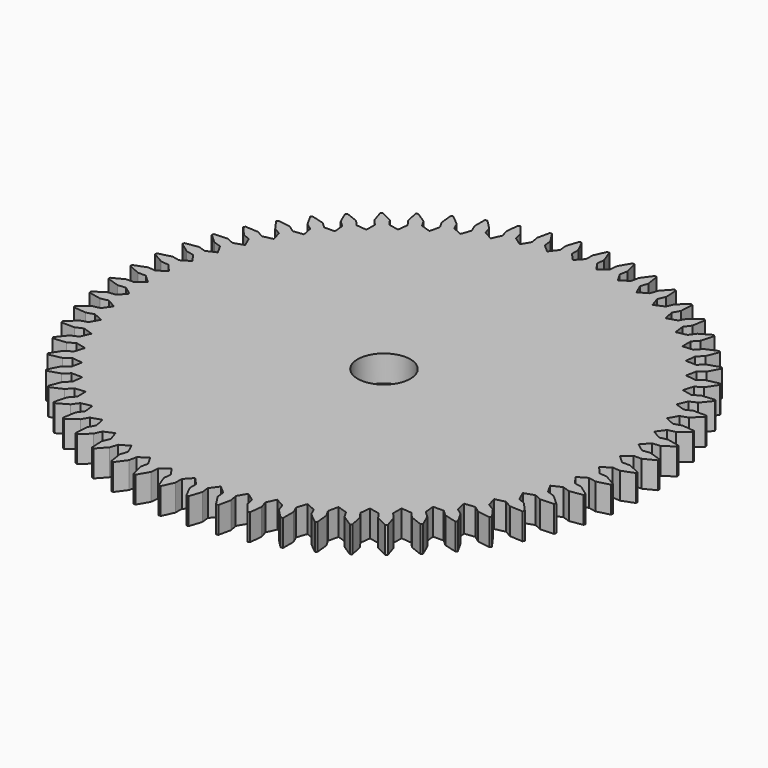
from build123d import *

# Parameters (mm, degrees)
F0_R            = 63.5
F1_DEPTH        = 6.35
F2_R            = 6.35
F3_DEPTH        = 25.4
F5_DEPTH        = 25.4
F5_COPIES_COUNT = 60


# Not quite as in the source:
# - a pattern or mirror of a feature is missing from the dataset's text; its kind, count and spacing are read off the source's solid


with BuildPart() as f1:
    # F0 (on Top) → F1 (new body)
    with BuildSketch(Plane.XY):
        Circle(F0_R)
    extrude(amount=F1_DEPTH)

    # F2 (on Top) → F3 (cut)
    with BuildSketch(Plane.XY):
        Circle(F2_R)
    extrude(amount=F3_DEPTH, mode=Mode.SUBTRACT)

    # F4 (on Top) → F5 (cut)
    with BuildSketch(Plane.XY):
        with BuildLine():
            Line((1.718201963, -60.5840606964), (1.718201963, -58.6790606964))
            Line((1.718201963, -58.6790606964), (0, -56.8083971739))
            Line((0, -56.8083971739), (-1.718201963, -58.6790606964))
            Line((-1.718201963, -58.6790606964), (-1.718201963, -60.5840606964))
            Line((-1.718201963, -60.5840606964), (-2.9970769528, -63.4217982329))
            add(Edge.make_bspline(
                [(-2.9970769528, -63.4217982329), (-2.0048973151, -63.9177481122), (0.0021103961, -64.9209688944), (2.093156251, -63.9252671778), (3.150477568, -63.4217982329)],
                knots=[0, 0, 0, 0, 0.494357661, 1, 1, 1, 1], degree=3))
            Line((3.150477568, -63.4217982329), (1.718201963, -60.5840606964))
        make_face()
    f5 = extrude(amount=F5_DEPTH, mode=Mode.SUBTRACT)

    # F5_copies: F5 ×60 about axis
    f5_copies_axis = Axis((0, 0, 0), (0, 0, 1))
    for i in range(1, F5_COPIES_COUNT):
        add(f5.rotate(f5_copies_axis, i * 360 / F5_COPIES_COUNT), mode=Mode.SUBTRACT)


solid = f1.part
